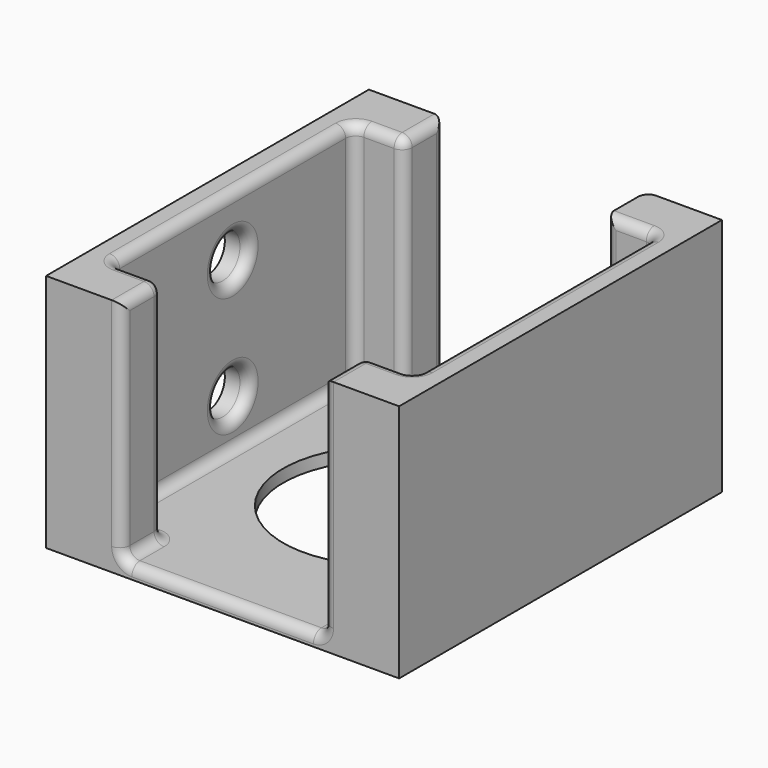
from build123d import *

# Parameters (mm, degrees)
F0_W      = 40
F0_H      = 40
F0_W_2    = 30
F0_H_2    = 30
F1_DEPTH  = 25
F2_W      = 20
F2_H      = 20
F3_DEPTH  = 40.001
F4_W      = 40
F4_H      = 40
F4_W_2    = 30
F4_H_2    = 30
F5_DEPTH  = 1.25
F6_R      = 10
F7_DEPTH  = 26.251
F9_DEPTH  = 40.001
F10_DEPTH = 2.5
F11_W     = 2.5
F11_H     = 40
F12_W     = 2.5
F12_H     = 40
F13_DEPTH = 23.751
F14_R     = 2.15
F15_DEPTH = 2.5
F16_R     = 1


with BuildPart() as f1:
    # F0 (on Top) → F1 (new body)
    with BuildSketch(Plane.XY):
        Rectangle(F0_W, F0_H)
        Rectangle(F0_W_2, F0_H_2, mode=Mode.SUBTRACT)
    extrude(amount=F1_DEPTH)

    # F2 (on face) → F3 (cut, through all)
    with BuildSketch(Plane.XZ.offset(20)):
        with Locations((0, 12.5)):
            Rectangle(F2_W, F2_H)
    extrude(amount=-F3_DEPTH, mode=Mode.SUBTRACT)

    # F4 (on face) → F5 (join)
    with BuildSketch(Plane(origin=(0, 0, 0), x_dir=(1, 0, 0), z_dir=(0, 0, -1))):
        Rectangle(F4_W, F4_H)
        Rectangle(F4_W_2, F4_H_2, mode=Mode.SUBTRACT)
        Rectangle(F4_W_2, F4_H_2)
    extrude(amount=F5_DEPTH)

    # F6 (on face) → F7 (cut, through all)
    with BuildSketch(Plane(origin=(0, 0, -1.25), x_dir=(1, 0, 0), z_dir=(0, 0, -1))):
        Circle(F6_R)
    extrude(amount=-F7_DEPTH, mode=Mode.SUBTRACT)

    # F8 (on face) → F9 (cut, through all)
    with BuildSketch(Plane.XZ.offset(20)):
        Polygon((-20, 25), (-20, 22.5), (-10, 22.5), (10, 22.5), (20, 22.5), (20, 25), align=None)
    extrude(amount=-F9_DEPTH, mode=Mode.SUBTRACT)

    # F10 (cut): faces of the model
    f10_faces = [f1.faces().sort_by_distance(p)[0] for p in [
        (0, 17.5, 2.5),
        (0, -17.5, 2.5),
    ]]
    extrude(f10_faces, amount=-F10_DEPTH, mode=Mode.SUBTRACT)

    # F11 (on face) + F12 (on face) → F13 (cut, through all)
    with BuildSketch(Plane.XY.offset(22.5)):
        with Locations((-18.75, 0)):
            Rectangle(F11_W, F11_H)
    with BuildSketch(Plane.XY.offset(22.5)):
        with Locations((18.75, 0)):
            Rectangle(F12_W, F12_H)
    extrude(amount=-F13_DEPTH, mode=Mode.SUBTRACT)

    # F14 (on face) → F15 (cut)
    with BuildSketch(Plane(origin=(-17.5, 0, 0), x_dir=(0, -1, 0), z_dir=(-1, 0, 0))):
        with Locations((0, 16.5625)):
            Circle(F14_R)
        with Locations((0, 4.6875)):
            Circle(F14_R)
    extrude(amount=-F15_DEPTH, mode=Mode.SUBTRACT)

    # F16
    f16_edges = [f1.edges().sort_by_distance(p)[0] for p in [
        (-10, -20, 11.25),
        (-10, -17.5, 0),
        (-10, -15, 11.25),
        (-10, -17.5, 22.5),
        (-10, 15, 11.25),
        (-10, 17.5, 22.5),
        (-10, 20, 11.25),
        (-10, 17.5, 0),
        (10, -20, 11.25),
        (10, -17.5, 0),
        (10, -15, 11.25),
        (10, -17.5, 22.5),
        (10, 17.5, 0),
        (12.5, 15, 0),
        (10, 15, 11.25),
        (12.5, 15, 22.5),
        (15, 15, 11.25),
        (15, 0, 0),
        (15, -15, 11.25),
        (15, 0, 22.5),
        (-15, 0, 0),
        (-15, -15, 11.25),
        (-15, 15, 11.25),
        (-15, 0, 22.5),
        (-15, 2.15, 16.5625),
        (-15, 2.15, 4.6875),
        (0, -20, 0),
        (12.5, -15, 22.5),
        (-12.5, -15, 0),
        (-12.5, 15, 0),
        (0, 20, 0),
        (12.5, -15, 0),
        (-12.5, -15, 22.5),
        (-12.5, 15, 22.5),
        (10, 20, 11.25),
    ]]
    fillet(f16_edges, radius=F16_R)


solid = f1.part
